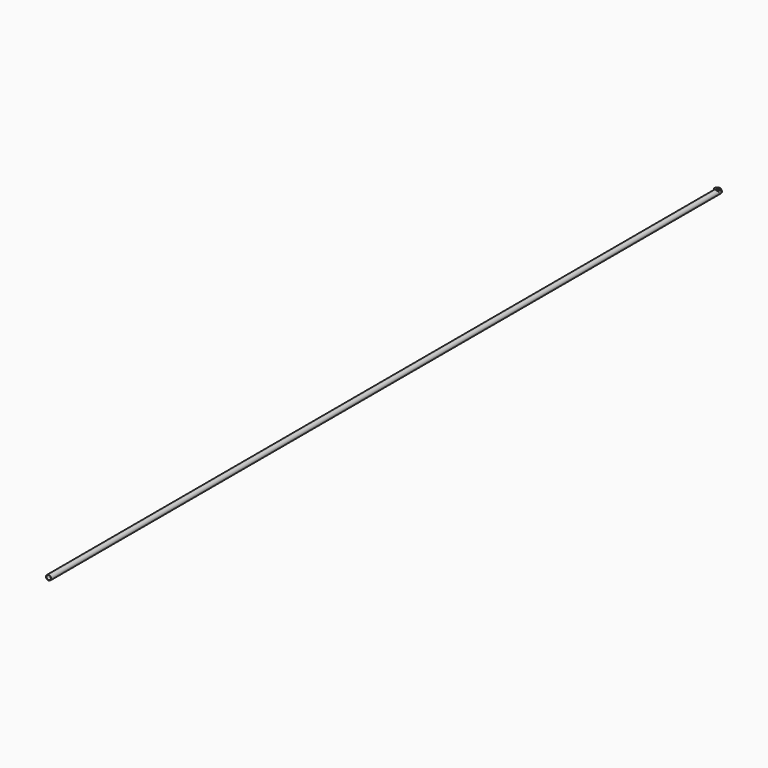
from build123d import *
from build123d import SkipClean  # not in build123d's __all__

# Parameters (mm, degrees)
F0_R     = 12.5
F1_DEPTH = 4075
F2_R     = 10.5
F3_DEPTH = 4050
F4_R     = 12.5
F5_DEPTH = 12.5
F6_R     = 10.5
F7_DEPTH = 12.5
F8_R     = 10.5
F9_DEPTH = 600


with BuildPart() as f1:
    # F0 (on Front) → F1 (new body)
    with BuildSketch(Plane.XZ):
        Circle(F0_R)
    extrude(amount=F1_DEPTH)

    # F2 (on face) → F3 (cut)
    with BuildSketch(Plane.XZ.offset(4075)):
        Circle(F2_R)
    extrude(amount=-F3_DEPTH, mode=Mode.SUBTRACT)

    # F4 (on Top) → F5 (join)
    with BuildSketch(Plane.XY):
        with Locations((0, -12.5)):
            Circle(F4_R)
    with SkipClean():  # cleaning this boolean's faces spoils the solid; the shape is the same uncleaned
        extrude(amount=F5_DEPTH)

    # F6 (on face) → F7 (cut)
    with BuildSketch(Plane.XY.offset(12.5)):
        with Locations((0, -12.5)):
            Circle(F6_R)
    with SkipClean():  # cleaning this boolean's faces spoils the solid; the shape is the same uncleaned
        extrude(amount=-F7_DEPTH, mode=Mode.SUBTRACT)

    # F8 (on Front) → F9 (cut)
    with BuildSketch(Plane.XZ):
        Circle(F8_R)
    with SkipClean():  # cleaning this boolean's faces spoils the solid; the shape is the same uncleaned
        extrude(amount=F9_DEPTH, mode=Mode.SUBTRACT)


solid = f1.part
